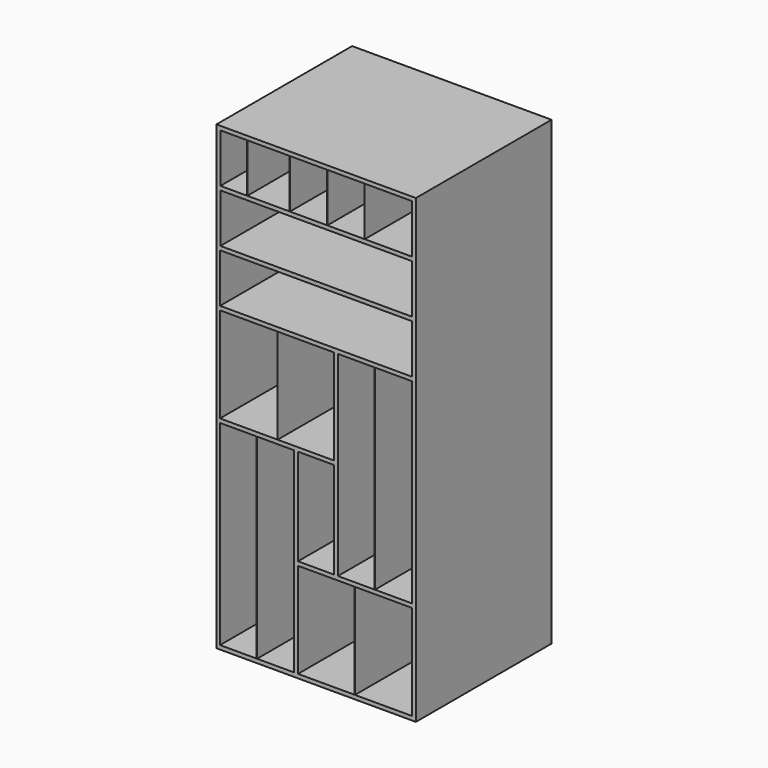
from build123d import *

# Parameters (mm, degrees)
F0_W     = 172.72
F0_H     = 19.05
F0_W_2   = 1.905
F0_H_2   = 939.8
F0_H_3   = 457.2
F0_H_4   = 234.95
F1_DEPTH = 812.8
F2_W     = 958.215
F2_H     = 2216.15
F3_DEPTH = 1.905


# Not quite as in the source:
# - a feature names something its author has since deleted; it is built from what else it names


with BuildPart() as f1:
    # F0 (on Front) → F1 (new body)
    with BuildSketch(Plane.XZ):
        Polygon((533.950886898, -1236.8191501617), (533.950886898, -1255.8691501617), (553.000886898, -1255.8691501617), (553.000886898, 960.2808498383), (533.950886898, 960.2808498383), (533.950886898, 941.2308498383), (533.950886898, 706.2808498383), (533.950886898, 687.2308498383), (533.950886898, 452.2808498383), (533.950886898, 433.2308498383), (533.950886898, 198.2808498383), (533.950886898, 179.2308498383), (533.950886898, -436.7191501617), (533.950886898, -760.5691501617), (533.950886898, -779.6191501617), align=None)
        Polygon((-212.174113102, -1236.8191501617), (-388.069113102, -1236.8191501617), (-388.069113102, -1255.8691501617), (-342.2091657827, -1255.8691501617), (532.045886898, -1255.8691501617), (533.950886898, -1255.8691501617), (533.950886898, -1236.8191501617), (532.045886898, -1236.8191501617), (260.265886898, -1236.8191501617), (258.360886898, -1236.8191501617), (-13.419113102, -1236.8191501617), (-32.469113102, -1236.8191501617), (-210.269113102, -1236.8191501617), align=None)
        Polygon((-388.069113102, -1255.8691501617), (-388.069113102, -1236.8191501617), (-388.069113102, -436.7191501617), (-388.069113102, -297.0191501617), (-388.069113102, -277.9691501617), (-388.069113102, 179.2308498383), (-388.069113102, 198.2808498383), (-388.069113102, 433.2308498383), (-388.069113102, 452.2808498383), (-386.164113102, 452.2808498383), (-386.164113102, 687.2308498383), (-386.164113102, 706.2808498383), (-386.164113102, 941.2308498383), (-259.164113102, 941.2308498383), (-257.259113102, 941.2308498383), (-54.059113102, 941.2308498383), (-52.154113102, 941.2308498383), (125.645886898, 941.2308498383), (127.550886898, 941.2308498383), (305.350886898, 941.2308498383), (307.255886898, 941.2308498383), (533.950886898, 941.2308498383), (533.950886898, 960.2808498383), (-282.659113102, 960.2808498383), (-405.214113102, 960.2808498383), (-405.214113102, -1255.8691501617), align=None)
        Polygon((-32.469113102, -297.0191501617), (-32.469113102, -1236.8191501617), (-13.419113102, -1236.8191501617), (-13.419113102, -779.6191501617), (-13.419113102, -760.5691501617), (-13.419113102, -297.0191501617), align=None)
        Polygon((-13.419113102, -760.5691501617), (-13.419113102, -779.6191501617), (258.360886898, -779.6191501617), (260.265886898, -779.6191501617), (533.950886898, -779.6191501617), (533.950886898, -760.5691501617), (356.150886898, -760.5691501617), (354.245886898, -760.5691501617), (178.350886898, -760.5691501617), (159.300886898, -760.5691501617), align=None)
        Polygon((159.300886898, -277.9691501617), (159.300886898, -297.0191501617), (159.300886898, -760.5691501617), (178.350886898, -760.5691501617), (178.350886898, 179.2308498383), (159.300886898, 179.2308498383), align=None)
        with Locations((72.940886898, -287.4941501617)):
            Rectangle(F0_W, F0_H)
        Polygon((-388.069113102, -297.0191501617), (-212.174113102, -297.0191501617), (-210.269113102, -297.0191501617), (-32.469113102, -297.0191501617), (-13.419113102, -297.0191501617), (-13.419113102, -277.9691501617), (-111.209113102, -277.9691501617), (-113.114113102, -277.9691501617), (-388.069113102, -277.9691501617), align=None)
        Polygon((-388.069113102, 198.2808498383), (-388.069113102, 179.2308498383), (-113.114113102, 179.2308498383), (-111.209113102, 179.2308498383), (159.300886898, 179.2308498383), (159.300886898, 198.2808498383), align=None)
        Polygon((533.950886898, 198.2808498383), (159.300886898, 198.2808498383), (159.300886898, 179.2308498383), (178.350886898, 179.2308498383), (354.245886898, 179.2308498383), (356.150886898, 179.2308498383), (533.950886898, 179.2308498383), align=None)
        Polygon((-388.069113102, 452.2808498383), (-388.069113102, 433.2308498383), (533.950886898, 433.2308498383), (533.950886898, 452.2808498383), (-386.164113102, 452.2808498383), align=None)
        Polygon((533.950886898, 687.2308498383), (533.950886898, 706.2808498383), (307.255886898, 706.2808498383), (305.350886898, 706.2808498383), (127.550886898, 706.2808498383), (125.645886898, 706.2808498383), (-52.154113102, 706.2808498383), (-54.059113102, 706.2808498383), (-257.259113102, 706.2808498383), (-259.164113102, 706.2808498383), (-386.164113102, 706.2808498383), (-386.164113102, 687.2308498383), align=None)
        with Locations((355.198386898, -290.6691501617)):
            Rectangle(F0_W_2, F0_H_2)
        with Locations((-112.161613102, -49.3691501617)):
            Rectangle(F0_W_2, F0_H_3)
        with Locations((-211.221613102, -766.9191501617)):
            Rectangle(F0_W_2, F0_H_2)
        with Locations((259.313386898, -1008.2191501617)):
            Rectangle(F0_W_2, F0_H_3)
        with Locations((-258.211613102, 823.7558498383)):
            Rectangle(F0_W_2, F0_H_4)
        with Locations((-53.106613102, 823.7558498383)):
            Rectangle(F0_W_2, F0_H_4)
        with Locations((126.598386898, 823.7558498383)):
            Rectangle(F0_W_2, F0_H_4)
        with Locations((306.303386898, 823.7558498383)):
            Rectangle(F0_W_2, F0_H_4)
    extrude(amount=F1_DEPTH)

    # F2 (on face) → F3 (join)
    with BuildSketch(Plane(origin=(0, 0, 0), x_dir=(-1, 0, 0), z_dir=(0, 1, 0))):
        with Locations((-73.893386898, -147.7941501617)):
            Rectangle(F2_W, F2_H)
    extrude(amount=F3_DEPTH)


solid = f1.part
